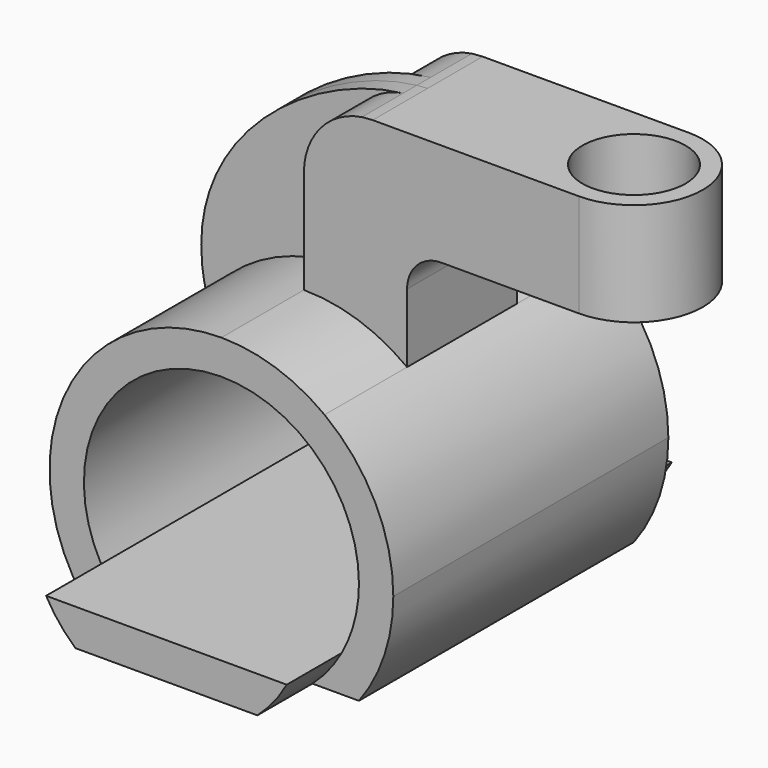
from build123d import *

# Parameters (mm, degrees)
F1_DEPTH      = 63.5
F0_W          = 25.4
F0_H          = 38.1
F2_DEPTH      = 25.4
F3_DEPTH      = 6.35
F4_ANGLE_BACK = 90
F4_ANGLE      = 180
F5_DEPTH      = 88.9
F6_R          = 19.05
F7_DEPTH      = 50.8


with BuildPart() as f1:
    # F0 (on Front) → F1 (new body, symmetric)
    with BuildSketch(Plane.XZ):
        with BuildLine():
            ThreePointArc((50.8, -38.1), (60.241389, -20.080463), (63.5, 0))
            ThreePointArc((63.5, 0), (56.796127, 28.398063), (38.1, 50.8))
            ThreePointArc((38.1, 50.8), (20.080463, 60.241389), (0, 63.5))
            ThreePointArc((0, 63.5), (-28.680443, 56.654057), (-51.176802, 37.592353))
            ThreePointArc((-51.176802, 37.592353), (-63.499213, -0.316103), (-50.8, -38.1))
            Line((-50.8, -38.1), (-33.601042, -38.1))
            ThreePointArc((-33.601042, -38.1), (-39.60553, -31.812607), (-44.45, -24.593444))
            ThreePointArc((-44.45, -24.593444), (-12.7, 49.186888), (50.8, 0))
            ThreePointArc((50.8, 0), (49.186888, -12.7), (44.45, -24.593444))
            ThreePointArc((44.45, -24.593444), (39.60553, -31.812607), (33.601042, -38.1))
            Line((33.601042, -38.1), (50.8, -38.1))
        make_face()
    extrude(amount=F1_DEPTH, both=True)

    # F0 (on Front) → F5 (join, symmetric)
    with BuildSketch(Plane.XZ):
        with BuildLine():
            Line((-33.601042, -38.1), (33.601042, -38.1))
            ThreePointArc((33.601042, -38.1), (39.60553, -31.812607), (44.45, -24.593444))
            Line((44.45, -24.593444), (-44.45, -24.593444))
            ThreePointArc((-44.45, -24.593444), (-39.60553, -31.812607), (-33.601042, -38.1))
        make_face()
    extrude(amount=F5_DEPTH, both=True)


with BuildPart() as f2:
    # F0 (on Front) → F2 (new body, symmetric)
    with BuildSketch(Plane.XZ):
        with BuildLine():
            ThreePointArc((0, 63.5), (20.080463, 60.241389), (38.1, 50.8))
            Line((38.1, 50.8), (38.1, 76.2))
            ThreePointArc((38.1, 76.2), (41.819744, 85.180256), (50.8, 88.9))
            Line((50.8, 88.9), (76.2, 88.9))
            Line((76.2, 88.9), (76.2, 127))
            Line((76.2, 127), (25.4, 127))
            add(Edge.make_bspline(
                [(25.4, 127), (24.082039, 126.940476), (22.740358, 126.833358), (21.379104, 126.679721)],
                knots=[0, 0, 0, 0, 4.313469, 4.313469, 4.313469, 4.313469], degree=3))
            ThreePointArc((21.379104, 126.679721), (6.070091, 118.077701), (0, 101.6))
            Line((0, 101.6), (0, 63.5))
        make_face()
        with Locations((88.9, 107.95)):
            Rectangle(F0_W, F0_H)
    extrude(amount=F2_DEPTH, both=True)

    # F0 (on Front) → F4 (revolve)
    with BuildSketch(Plane.XZ, mode=Mode.PRIVATE) as f4_sk:
        with Locations((114.3, 107.95)):
            Rectangle(F0_W, F0_H)
    revolve(f4_sk.sketch.rotate(Axis((101.6, 0, 107.95), (0, 0, -1)), -F4_ANGLE_BACK), axis=Axis((101.6, 0, 107.95), (0, 0, -1)), revolution_arc=F4_ANGLE)

    # F6 (on face) → F7 (cut)
    with BuildSketch(Plane.XY.offset(127)):
        with Locations((101.6, 0)):
            Circle(F6_R)
    extrude(amount=-F7_DEPTH, mode=Mode.SUBTRACT)


with BuildPart() as f3:
    # F0 (on Front) → F3 (new body, symmetric)
    with BuildSketch(Plane.XZ):
        with BuildLine():
            ThreePointArc((-51.176802, 37.592353), (-28.680443, 56.654057), (0, 63.5))
            Line((0, 63.5), (0, 101.6))
            ThreePointArc((0, 101.6), (6.070091, 118.077701), (21.379104, 126.679721))
            add(Edge.make_bspline(
                [(21.379104, 126.679721), (-14.40962, 122.640434), (-63.7269, 86.445565), (-51.176802, 37.592353)],
                knots=[4.313469, 4.313469, 4.313469, 4.313469, 117.718877, 117.718877, 117.718877, 117.718877], degree=3))
        make_face()
    extrude(amount=F3_DEPTH, both=True)


solid = Compound([f1.part, f2.part, f3.part])
